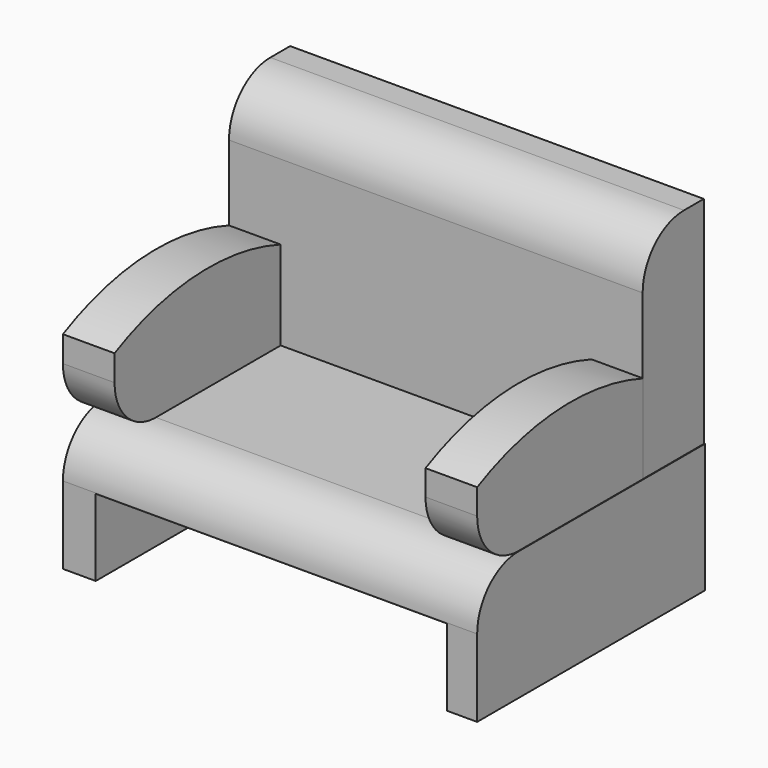
from build123d import *

# Parameters (mm, degrees)
F0_W      = 80.2132
F0_H      = 55.1688
F1_DEPTH  = 25
F3_W      = 80.0983905792
F3_H      = 66.7644366622
F4_DEPTH  = 14.8
F6_DEPTH  = 10
F9_DEPTH  = 10
F10_W     = 67.9705310613
F10_H     = 14.8716745898
F11_DEPTH = 99
F12_R     = 10
F12_2_R   = 10
F12_3_R   = 10


with BuildPart() as f1:
    # F0 (on Top) → F1 (new body)
    with BuildSketch(Plane.XY):
        with Locations((40.1066, 27.5844)):
            Rectangle(F0_W, F0_H)
    extrude(amount=F1_DEPTH)

    # F3 (on offset) → F4 (join)
    with BuildSketch(Plane.XZ.offset(-55)):
        with Locations((40.0491952896, 33.3822183311)):
            Rectangle(F3_W, F3_H)
    extrude(amount=F4_DEPTH)

    # F10 (on Front) → F11 (cut)
    with BuildSketch(Plane.XZ):
        with Locations((40.3414806351, 7.4358372949)):
            Rectangle(F10_W, F10_H)
    extrude(amount=-F11_DEPTH, mode=Mode.SUBTRACT)

    # F12
    f12_edges = [f1.edges().sort_by_distance(p)[0] for p in [
        (40.1066, 0, 25),
        (40.049195, 40.2, 66.764437),
    ]]
    fillet(f12_edges, radius=F12_R)


with BuildPart() as f6:
    # F5 (on Right) → F6 (new body)
    with BuildSketch(Plane.YZ):
        with BuildLine():
            Line((40.1999726892, 24.9999165535), (40.1999726892, 42.2092106919))
            ThreePointArc((40.1999726892, 42.2092106919), (19.8718728741, 45.2787326204), (0, 40.0097407401))
            Line((0, 40.0097407401), (0, 24.9999165535))
            Line((0, 24.9999165535), (40.1999726892, 24.9999165535))
        make_face()
    extrude(amount=F6_DEPTH)

    # F12#2
    f12_2_edges = [f6.edges().sort_by_distance(p)[0] for p in [
        (5, 0, 24.999917),
    ]]
    fillet(f12_2_edges, radius=F12_2_R)


with BuildPart() as f9:
    # F8 (on offset) → F9 (new body)
    with BuildSketch(Plane.YZ.offset(70.213)):
        with BuildLine():
            Line((40.1988625526, 25.079857558), (40.1999279857, 42.2091931105))
            ThreePointArc((40.1999279857, 42.2091931105), (19.8724426746, 45.2681878924), (0, 40.0098487735))
            Line((0, 40.0098487735), (0, 25.079857558))
            Line((0, 25.079857558), (40.1988625526, 25.079857558))
        make_face()
    extrude(amount=F9_DEPTH)

    # F12#3
    f12_3_edges = [f9.edges().sort_by_distance(p)[0] for p in [
        (75.213, 0, 25.079858),
    ]]
    fillet(f12_3_edges, radius=F12_3_R)


solid = Compound([f1.part, f6.part, f9.part])
